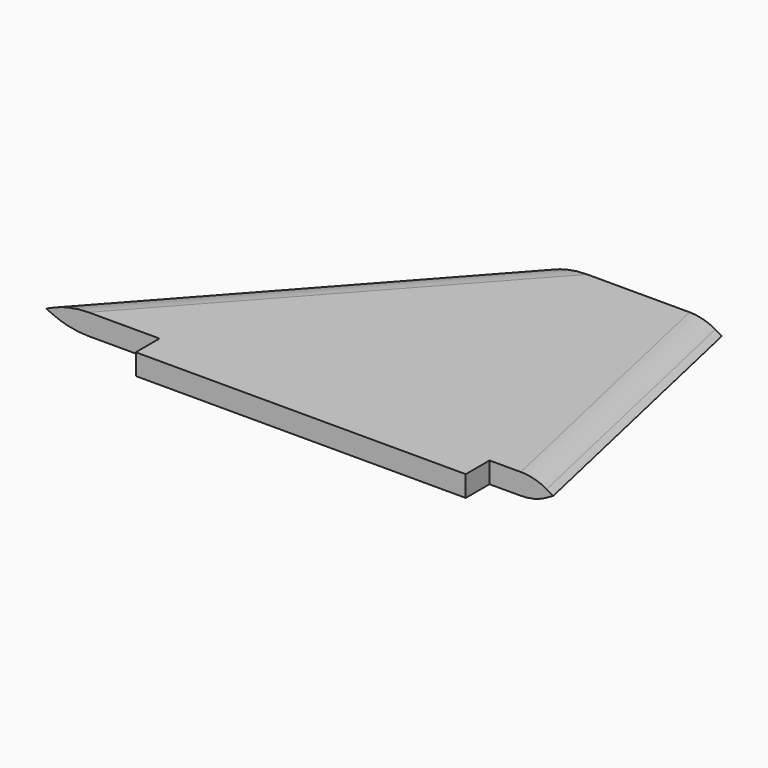
from build123d import *

# Parameters (mm, degrees)
F0_W        = 50
F0_H        = 4.5
F1_DEPTH    = 1.5875
F2_T1_DEPTH = 84.8335063877
F3_T1_DEPTH = 61.4898569594
F4_R        = 7.62


# Not quite as in the source:
# - a fillet or chamfer that OpenCascade refuses, or shapes differently, is made with other operations: its cross-section is extruded or revolved along the edge and cut away or added


with BuildPart() as f1:
    # F0 (on Top) → F1 (new body, symmetric)
    with BuildSketch(Plane.XY):
        Polygon((40, 44.444437807), (0, 0), (20, 0), (70, 0), (80, 0), (70, 44.444437807), align=None)
        with Locations((45, -2.25)):
            Rectangle(F0_W, F0_H)
    extrude(amount=F1_DEPTH, both=True)

    # F2: chamfer of 2.794 x 4.8393499563 on 2 edges, made by hand

    # F2_s2 → F2_t1 (cut)
    with BuildSketch(Plane(origin=(48.3753142579, 53.7503411482, 0), x_dir=(0, 0, 1), z_dir=(-0.6689647868, -0.7432940966, 0))):
        Polygon((1.2065, 0), (-1.5875, -4.8393499563), (-1.5875, 0), align=None)
        Polygon((-1.2065, 0), (1.5875, -4.8393499563), (1.5875, 0), align=None)
    extrude(amount=F2_T1_DEPTH, mode=Mode.SUBTRACT)

    # F3: chamfer of 1.778 x 3.0795863359 on 2 edges, made by hand

    # F3_s2 → F3_t1 (cut)
    with BuildSketch(Plane(origin=(5.6037370993, -24.9054944995, 0), x_dir=(0, 0, 1), z_dir=(-0.2195122263, 0.9756097491, 0))):
        Polygon((-1.5875, 74.9691935903), (0.1905, 78.0487799262), (-1.5875, 78.0487799262), align=None)
        Polygon((-0.1905, 78.0487799262), (1.5875, 74.9691935903), (1.5875, 78.0487799262), align=None)
    extrude(amount=F3_T1_DEPTH, mode=Mode.SUBTRACT)

    # F4
    f4_edges = [f1.edges().sort_by_distance(p)[0] for p in [
        (26.51068, 22.222219, -1.5875),
        (71.843424, 22.222219, -1.5875),
        (71.843424, 22.222219, 1.5875),
        (26.51068, 22.222219, 1.5875),
    ]]
    fillet(f4_edges, radius=F4_R)


solid = f1.part
